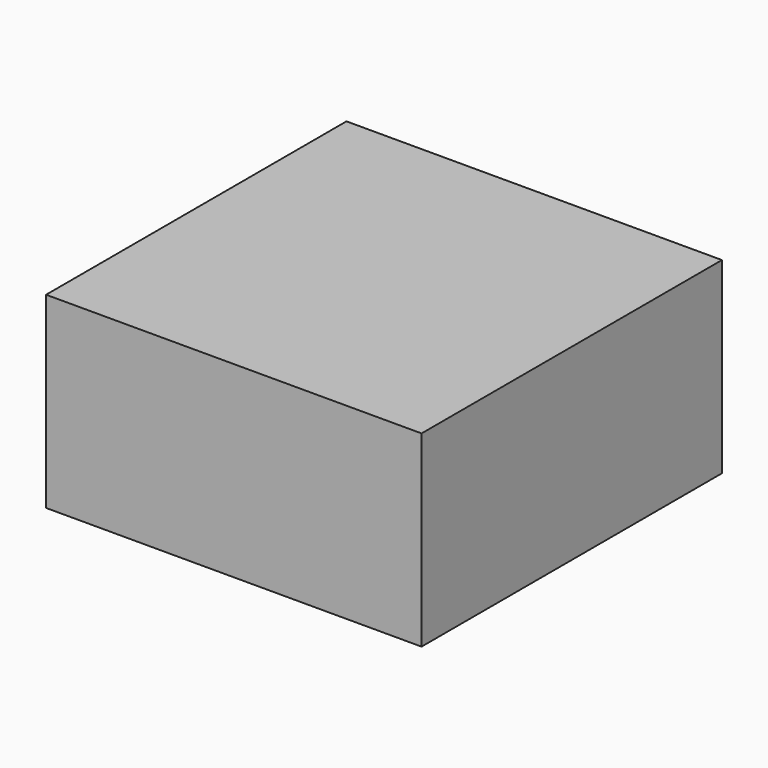
from build123d import *

# Parameters (mm, degrees)
F0_W     = 20
F0_H     = 20
F1_DEPTH = 10
F2_T     = -1


# Not quite as in the source:
# - a feature names something its author has since deleted; it is built from what else it names


with BuildPart() as f1:
    # F0 (on Top) → F1 (new body)
    with BuildSketch(Plane.XY):
        Rectangle(F0_W, F0_H)
    extrude(amount=F1_DEPTH)

    # F2 (hollow: no face is removed)
    offset(amount=F2_T, mode=Mode.SUBTRACT)


solid = f1.part
